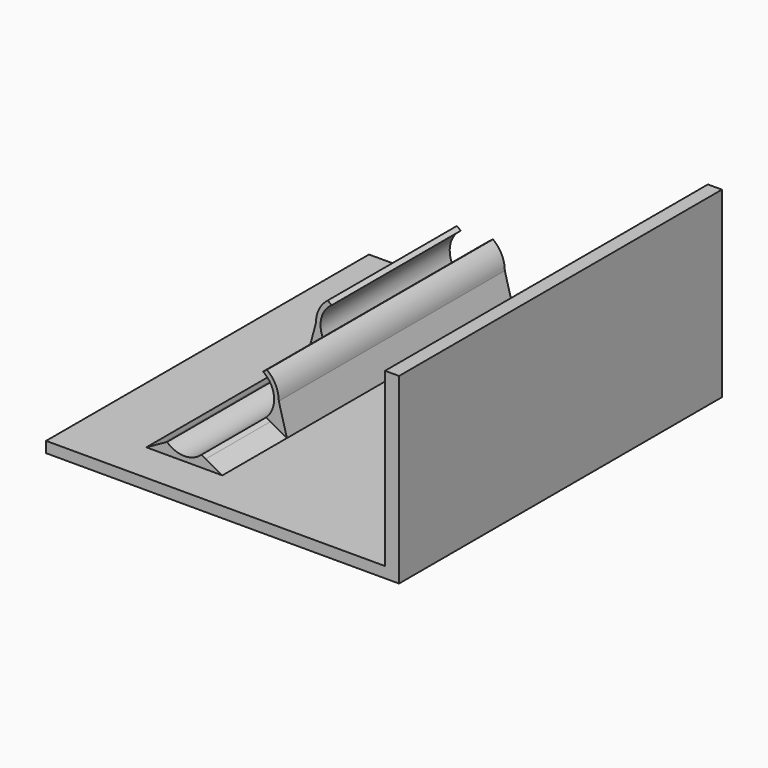
from build123d import *

# Parameters (mm, degrees)
F1_DEPTH = 90
F2_DEPTH = 40
F0_W     = 3.4774128616
F0_H     = 42.5927758359
F3_DEPTH = 100
F4_DEPTH = 70


# Not quite as in the source:
# - a feature names something its author has since deleted; it is built from what else it names


with BuildPart() as f1:
    # F0 (on Front) → F1 (new body)
    with BuildSketch(Plane.XZ):
        with BuildLine():
            ThreePointArc((4.2720749172, -4.5620034965), (0, -6.25), (-4.2720749172, -4.5620034965))
            Line((-4.2720749172, -4.5620034965), (-5.3278356976, -5.1455675625))
            ThreePointArc((-5.3278356976, -5.1455675625), (-2.8939428024, -6.818195789), (0, -7.4069358551))
            ThreePointArc((0, -7.4069358551), (2.8939428024, -6.818195789), (5.3278356976, -5.1455675625))
            Line((5.3278356976, -5.1455675625), (4.2720749172, -4.5620034965))
        make_face()
        with BuildLine():
            Line((9.4190128148, -7.4069358551), (5.3278356976, -5.1455675625))
            ThreePointArc((5.3278356976, -5.1455675625), (2.8939428024, -6.818195789), (0, -7.4069358551))
            Line((0, -7.4069358551), (9.4190128148, -7.4069358551))
        make_face()
        with BuildLine():
            ThreePointArc((0, -7.4069358551), (-2.8939428024, -6.818195789), (-5.3278356976, -5.1455675625))
            Line((-5.3278356976, -5.1455675625), (-9.4190128148, -7.4069358551))
            Line((-9.4190128148, -7.4069358551), (0, -7.4069358551))
        make_face()
        Polygon((9.4190128148, -7.4069358551), (0, -7.4069358551), (0, -10.1), (61.2, -10.1), (61.2, -7.4069358551), (57.7225871384, -7.4069358551), align=None)
    extrude(amount=F1_DEPTH)

    # F0 (on Front) → F2 (join)
    with BuildSketch(Plane.XZ):
        with BuildLine():
            Line((-9.4190128148, -7.4069358551), (-5.3278356976, -5.1455675625))
            ThreePointArc((-5.3278356976, -5.1455675625), (-6.8675190578, -2.7748658979), (-7.4069358551, 0))
            Line((-7.4069358551, 0), (-9.4190128148, -7.4069358551))
        make_face()
        with BuildLine():
            ThreePointArc((-4.2720749172, -4.5620034965), (-6.230456475, 0.4938745919), (-3.5, 5.1780787943))
            Line((-3.5, 5.1780787943), (-4.4709416805, 5.9053686803))
            ThreePointArc((-4.4709416805, 5.9053686803), (-6.6324458912, 3.2974778636), (-7.4069358551, 0))
            ThreePointArc((-7.4069358551, 0), (-6.8675190578, -2.7748658979), (-5.3278356976, -5.1455675625))
            Line((-5.3278356976, -5.1455675625), (-4.2720749172, -4.5620034965))
        make_face()
        with BuildLine():
            ThreePointArc((3.5, 5.1780787943), (6.230456475, 0.4938745919), (4.2720749172, -4.5620034965))
            Line((4.2720749172, -4.5620034965), (5.3278356976, -5.1455675625))
            ThreePointArc((5.3278356976, -5.1455675625), (6.8675190578, -2.7748658979), (7.4069358551, 0))
            ThreePointArc((7.4069358551, 0), (6.6324458912, 3.2974778636), (4.4709416805, 5.9053686803))
            Line((4.4709416805, 5.9053686803), (3.5, 5.1780787943))
        make_face()
        with BuildLine():
            ThreePointArc((7.4069358551, 0), (6.8675190578, -2.7748658979), (5.3278356976, -5.1455675625))
            Line((5.3278356976, -5.1455675625), (9.4190128148, -7.4069358551))
            Line((9.4190128148, -7.4069358551), (7.4069358551, 0))
        make_face()
    extrude(amount=F2_DEPTH)

    # F0 (on Front) → F3 (join)
    with BuildSketch(Plane.XZ):
        Polygon((0, -10.1), (0, -7.4069358551), (-9.4190128148, -7.4069358551), (-26.2554790825, -7.4069358551), (-26.2554790825, -10.1), align=None)
        Polygon((9.4190128148, -7.4069358551), (0, -7.4069358551), (0, -10.1), (61.2, -10.1), (61.2, -7.4069358551), (57.7225871384, -7.4069358551), align=None)
        with Locations((59.4612935692, 13.8894520629)):
            Rectangle(F0_W, F0_H)
    extrude(amount=F3_DEPTH)

    # F0 (on Front) → F4 (join)
    with BuildSketch(Plane.XZ):
        with BuildLine():
            ThreePointArc((3.5, 5.1780787943), (6.230456475, 0.4938745919), (4.2720749172, -4.5620034965))
            Line((4.2720749172, -4.5620034965), (5.3278356976, -5.1455675625))
            ThreePointArc((5.3278356976, -5.1455675625), (6.8675190578, -2.7748658979), (7.4069358551, 0))
            ThreePointArc((7.4069358551, 0), (6.6324458912, 3.2974778636), (4.4709416805, 5.9053686803))
            Line((4.4709416805, 5.9053686803), (3.5, 5.1780787943))
        make_face()
        with BuildLine():
            ThreePointArc((7.4069358551, 0), (6.8675190578, -2.7748658979), (5.3278356976, -5.1455675625))
            Line((5.3278356976, -5.1455675625), (9.4190128148, -7.4069358551))
            Line((9.4190128148, -7.4069358551), (7.4069358551, 0))
        make_face()
    extrude(amount=F4_DEPTH)


solid = f1.part
